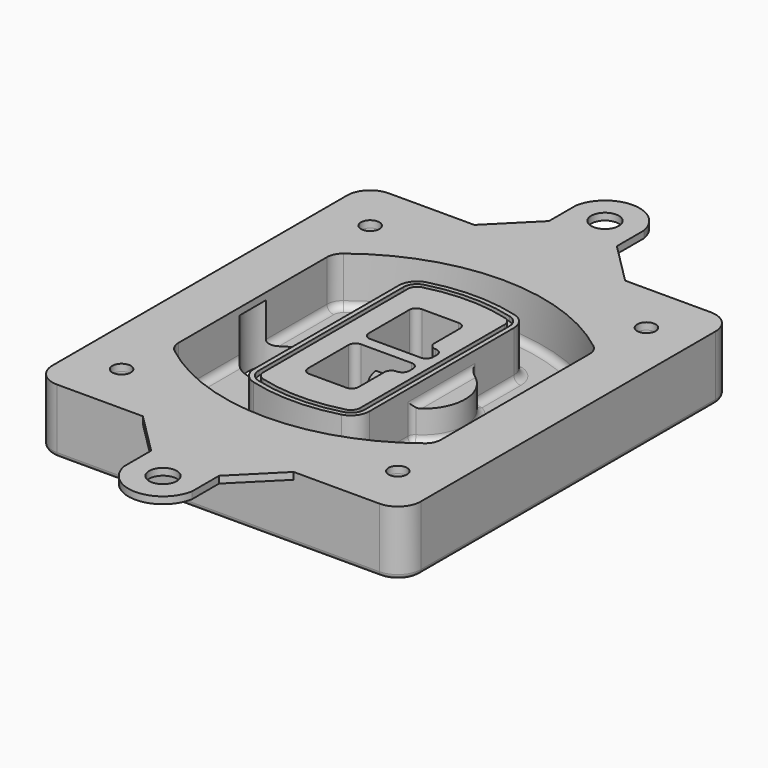
from build123d import *

# Parameters (mm, degrees)
F0_R      = 4
F1_DEPTH  = 25
F2_DEPTH  = 3
F3_DEPTH  = 18
F5_DEPTH  = 21
F6_DEPTH  = 2
F8_DEPTH  = 20
F9_DEPTH  = 16
F10_DEPTH = 25
F7_R      = 6
F7_R_2    = 4
F11_DEPTH = 6
F13_DEPTH = 9
F14_R     = 3
F15_R     = 2
F16_R     = 4
F16_R_2   = 6
F17_DEPTH = 3


# Not quite as in the source:
# - a feature names something its author has since deleted; it is built from what else it names


with BuildPart() as f1:
    # F0 (on Top) → F1 (new body)
    with BuildSketch(Plane.XY):
        with BuildLine():
            ThreePointArc((-80, -80), (-77.0710678119, -87.0710678119), (-70, -90))
            Line((-70, -90), (70, -90))
            ThreePointArc((70, -90), (77.0710678119, -87.0710678119), (80, -80))
            Line((80, -80), (80, 80))
            ThreePointArc((80, 80), (77.0710678119, 87.0710678119), (70, 90))
            Line((70, 90), (-70, 90))
            ThreePointArc((-70, 90), (-77.0710678119, 87.0710678119), (-80, 80))
            Line((-80, 80), (-80, -80))
        make_face()
        with Locations((-60, -67.5)):
            Circle(F0_R, mode=Mode.SUBTRACT)
        with Locations((60, -67.5)):
            Circle(F0_R, mode=Mode.SUBTRACT)
        with Locations((-60, 67.5)):
            Circle(F0_R, mode=Mode.SUBTRACT)
        with BuildLine():
            ThreePointArc((-64, 40.2934422872), (-62.5820384798, 46.4328484224), (-58.6153846154, 51.3286200352))
            ThreePointArc((-58.6153846154, 51.3286200352), (0, 71.5), (58.6153846154, 51.3286200352))
            ThreePointArc((58.6153846154, 51.3286200352), (62.5820384798, 46.4328484224), (64, 40.2934422872))
            Line((64, 40.2934422872), (64, -40.2934422872))
            ThreePointArc((64, -40.2934422872), (62.5820384798, -46.4328484224), (58.6153846154, -51.3286200352))
            ThreePointArc((58.6153846154, -51.3286200352), (0, -71.5), (-58.6153846154, -51.3286200352))
            ThreePointArc((-58.6153846154, -51.3286200352), (-62.5820384798, -46.4328484224), (-64, -40.2934422872))
            Line((-64, -40.2934422872), (-64, 40.2934422872))
        make_face(mode=Mode.SUBTRACT)
        with Locations((60, 67.5)):
            Circle(F0_R, mode=Mode.SUBTRACT)
        with BuildLine():
            ThreePointArc((58.6153846154, 51.3286200352), (0, 71.5), (-58.6153846154, 51.3286200352))
            ThreePointArc((-58.6153846154, 51.3286200352), (-62.5820384798, 46.4328484224), (-64, 40.2934422872))
            Line((-64, 40.2934422872), (-64, -40.2934422872))
            ThreePointArc((-64, -40.2934422872), (-62.5820384798, -46.4328484224), (-58.6153846154, -51.3286200352))
            ThreePointArc((-58.6153846154, -51.3286200352), (0, -71.5), (58.6153846154, -51.3286200352))
            ThreePointArc((58.6153846154, -51.3286200352), (62.5820384798, -46.4328484224), (64, -40.2934422872))
            Line((64, -40.2934422872), (64, 40.2934422872))
            ThreePointArc((64, 40.2934422872), (62.5820384798, 46.4328484224), (58.6153846154, 51.3286200352))
        make_face()
        with BuildLine():
            Line((-60, -40.2934422872), (-60, 40.2934422872))
            ThreePointArc((-60, 40.2934422872), (-58.9871703427, 44.6787323838), (-56.1538461538, 48.1757121072))
            ThreePointArc((-56.1538461538, 48.1757121072), (0, 67.5), (56.1538461538, 48.1757121072))
            ThreePointArc((56.1538461538, 48.1757121072), (58.9871703427, 44.6787323838), (60, 40.2934422872))
            Line((60, 40.2934422872), (60, -40.2934422872))
            ThreePointArc((60, -40.2934422872), (58.9871703427, -44.6787323838), (56.1538461538, -48.1757121072))
            ThreePointArc((56.1538461538, -48.1757121072), (0, -67.5), (-56.1538461538, -48.1757121072))
            ThreePointArc((-56.1538461538, -48.1757121072), (-58.9871703427, -44.6787323838), (-60, -40.2934422872))
        make_face(mode=Mode.SUBTRACT)
        with BuildLine():
            ThreePointArc((-56.1538461538, 48.1757121072), (-58.9871703427, 44.6787323838), (-60, 40.2934422872))
            Line((-60, 40.2934422872), (-60, -40.2934422872))
            ThreePointArc((-60, -40.2934422872), (-58.9871703427, -44.6787323838), (-56.1538461538, -48.1757121072))
            ThreePointArc((-56.1538461538, -48.1757121072), (0, -67.5), (56.1538461538, -48.1757121072))
            ThreePointArc((56.1538461538, -48.1757121072), (58.9871703427, -44.6787323838), (60, -40.2934422872))
            Line((60, -40.2934422872), (60, 40.2934422872))
            ThreePointArc((60, 40.2934422872), (58.9871703427, 44.6787323838), (56.1538461538, 48.1757121072))
            ThreePointArc((56.1538461538, 48.1757121072), (0, 67.5), (-56.1538461538, 48.1757121072))
        make_face()
        with BuildLine():
            ThreePointArc((54.3076923077, 45.8110311612), (56.2910192399, 43.3631453548), (57, 40.2934422872))
            Line((57, 40.2934422872), (57, -40.2934422872))
            ThreePointArc((57, -40.2934422872), (56.2910192399, -43.3631453548), (54.3076923077, -45.8110311612))
            ThreePointArc((54.3076923077, -45.8110311612), (0, -64.5), (-54.3076923077, -45.8110311612))
            ThreePointArc((-54.3076923077, -45.8110311612), (-56.2910192399, -43.3631453548), (-57, -40.2934422872))
            Line((-57, -40.2934422872), (-57, 40.2934422872))
            ThreePointArc((-57, 40.2934422872), (-56.2910192399, 43.3631453548), (-54.3076923077, 45.8110311612))
            ThreePointArc((-54.3076923077, 45.8110311612), (0, 64.5), (54.3076923077, 45.8110311612))
        make_face(mode=Mode.SUBTRACT)
        with BuildLine():
            Line((57, -40.2934422872), (57, 40.2934422872))
            ThreePointArc((57, 40.2934422872), (56.2910192399, 43.3631453548), (54.3076923077, 45.8110311612))
            ThreePointArc((54.3076923077, 45.8110311612), (0, 64.5), (-54.3076923077, 45.8110311612))
            ThreePointArc((-54.3076923077, 45.8110311612), (-56.2910192399, 43.3631453548), (-57, 40.2934422872))
            Line((-57, 40.2934422872), (-57, -40.2934422872))
            ThreePointArc((-57, -40.2934422872), (-56.2910192399, -43.3631453548), (-54.3076923077, -45.8110311612))
            ThreePointArc((-54.3076923077, -45.8110311612), (0, -64.5), (54.3076923077, -45.8110311612))
            ThreePointArc((54.3076923077, -45.8110311612), (56.2910192399, -43.3631453548), (57, -40.2934422872))
        make_face()
    extrude(amount=-F1_DEPTH)

    # F0 (on Top) → F2 (join)
    with BuildSketch(Plane.XY):
        with BuildLine():
            ThreePointArc((-56.1538461538, 48.1757121072), (-58.9871703427, 44.6787323838), (-60, 40.2934422872))
            Line((-60, 40.2934422872), (-60, -40.2934422872))
            ThreePointArc((-60, -40.2934422872), (-58.9871703427, -44.6787323838), (-56.1538461538, -48.1757121072))
            ThreePointArc((-56.1538461538, -48.1757121072), (0, -67.5), (56.1538461538, -48.1757121072))
            ThreePointArc((56.1538461538, -48.1757121072), (58.9871703427, -44.6787323838), (60, -40.2934422872))
            Line((60, -40.2934422872), (60, 40.2934422872))
            ThreePointArc((60, 40.2934422872), (58.9871703427, 44.6787323838), (56.1538461538, 48.1757121072))
            ThreePointArc((56.1538461538, 48.1757121072), (0, 67.5), (-56.1538461538, 48.1757121072))
        make_face()
        with BuildLine():
            ThreePointArc((54.3076923077, 45.8110311612), (56.2910192399, 43.3631453548), (57, 40.2934422872))
            Line((57, 40.2934422872), (57, -40.2934422872))
            ThreePointArc((57, -40.2934422872), (56.2910192399, -43.3631453548), (54.3076923077, -45.8110311612))
            ThreePointArc((54.3076923077, -45.8110311612), (0, -64.5), (-54.3076923077, -45.8110311612))
            ThreePointArc((-54.3076923077, -45.8110311612), (-56.2910192399, -43.3631453548), (-57, -40.2934422872))
            Line((-57, -40.2934422872), (-57, 40.2934422872))
            ThreePointArc((-57, 40.2934422872), (-56.2910192399, 43.3631453548), (-54.3076923077, 45.8110311612))
            ThreePointArc((-54.3076923077, 45.8110311612), (0, 64.5), (54.3076923077, 45.8110311612))
        make_face(mode=Mode.SUBTRACT)
    extrude(amount=F2_DEPTH)

    # F0 (on Top) → F3 (cut)
    with BuildSketch(Plane.XY):
        with BuildLine():
            Line((57, -40.2934422872), (57, 40.2934422872))
            ThreePointArc((57, 40.2934422872), (56.2910192399, 43.3631453548), (54.3076923077, 45.8110311612))
            ThreePointArc((54.3076923077, 45.8110311612), (0, 64.5), (-54.3076923077, 45.8110311612))
            ThreePointArc((-54.3076923077, 45.8110311612), (-56.2910192399, 43.3631453548), (-57, 40.2934422872))
            Line((-57, 40.2934422872), (-57, -40.2934422872))
            ThreePointArc((-57, -40.2934422872), (-56.2910192399, -43.3631453548), (-54.3076923077, -45.8110311612))
            ThreePointArc((-54.3076923077, -45.8110311612), (0, -64.5), (54.3076923077, -45.8110311612))
            ThreePointArc((54.3076923077, -45.8110311612), (56.2910192399, -43.3631453548), (57, -40.2934422872))
        make_face()
    extrude(amount=-F3_DEPTH, mode=Mode.SUBTRACT)

    # F4 (on face) → F5 (join, through all)
    with BuildSketch(Plane.XY.offset(3)):
        with BuildLine():
            ThreePointArc((-25, -39.2465276821), (-23.3511545998, -44.1109737193), (-19.0842911877, -46.9702398883))
            ThreePointArc((-19.0842911877, -46.9702398883), (0, -49.5), (19.0842911877, -46.9702398883))
            ThreePointArc((19.0842911877, -46.9702398883), (23.3511545998, -44.1109737193), (25, -39.2465276821))
            Line((25, -39.2465276821), (25, 39.2465276821))
            ThreePointArc((25, 39.2465276821), (23.3511545998, 44.1109737193), (19.0842911877, 46.9702398883))
            ThreePointArc((19.0842911877, 46.9702398883), (0, 49.5), (-19.0842911877, 46.9702398883))
            ThreePointArc((-19.0842911877, 46.9702398883), (-23.3511545998, 44.1109737193), (-25, 39.2465276821))
            Line((-25, 39.2465276821), (-25, -39.2465276821))
        make_face()
        with BuildLine():
            ThreePointArc((18.5632183908, 45.0393118368), (21.7633659499, 42.89486221), (23, 39.2465276821))
            Line((23, 39.2465276821), (23, -39.2465276821))
            ThreePointArc((23, -39.2465276821), (21.7633659499, -42.89486221), (18.5632183908, -45.0393118368))
            ThreePointArc((18.5632183908, -45.0393118368), (0, -47.5), (-18.5632183908, -45.0393118368))
            ThreePointArc((-18.5632183908, -45.0393118368), (-21.7633659499, -42.89486221), (-23, -39.2465276821))
            Line((-23, -39.2465276821), (-23, 39.2465276821))
            ThreePointArc((-23, 39.2465276821), (-21.7633659499, 42.89486221), (-18.5632183908, 45.0393118368))
            ThreePointArc((-18.5632183908, 45.0393118368), (0, 47.5), (18.5632183908, 45.0393118368))
        make_face(mode=Mode.SUBTRACT)
        with BuildLine():
            Line((23, -39.2465276821), (23, 39.2465276821))
            ThreePointArc((23, 39.2465276821), (21.7633659499, 42.89486221), (18.5632183908, 45.0393118368))
            ThreePointArc((18.5632183908, 45.0393118368), (0, 47.5), (-18.5632183908, 45.0393118368))
            ThreePointArc((-18.5632183908, 45.0393118368), (-21.7633659499, 42.89486221), (-23, 39.2465276821))
            Line((-23, 39.2465276821), (-23, -39.2465276821))
            ThreePointArc((-23, -39.2465276821), (-21.7633659499, -42.89486221), (-18.5632183908, -45.0393118368))
            ThreePointArc((-18.5632183908, -45.0393118368), (0, -47.5), (18.5632183908, -45.0393118368))
            ThreePointArc((18.5632183908, -45.0393118368), (21.7633659499, -42.89486221), (23, -39.2465276821))
        make_face()
        with BuildLine():
            ThreePointArc((18.0421455939, 43.1083837852), (20.1755772999, 41.6787507007), (21, 39.2465276821))
            Line((21, 39.2465276821), (21, -39.2465276821))
            ThreePointArc((21, -39.2465276821), (20.1755772999, -41.6787507007), (18.0421455939, -43.1083837852))
            ThreePointArc((18.0421455939, -43.1083837852), (0, -45.5), (-18.0421455939, -43.1083837852))
            ThreePointArc((-18.0421455939, -43.1083837852), (-20.1755772999, -41.6787507007), (-21, -39.2465276821))
            Line((-21, -39.2465276821), (-21, 39.2465276821))
            ThreePointArc((-21, 39.2465276821), (-20.1755772999, 41.6787507007), (-18.0421455939, 43.1083837852))
            ThreePointArc((-18.0421455939, 43.1083837852), (0, 45.5), (18.0421455939, 43.1083837852))
        make_face(mode=Mode.SUBTRACT)
        with BuildLine():
            Line((21, -39.2465276821), (21, 39.2465276821))
            ThreePointArc((21, 39.2465276821), (20.1755772999, 41.6787507007), (18.0421455939, 43.1083837852))
            ThreePointArc((18.0421455939, 43.1083837852), (0, 45.5), (-18.0421455939, 43.1083837852))
            ThreePointArc((-18.0421455939, 43.1083837852), (-20.1755772999, 41.6787507007), (-21, 39.2465276821))
            Line((-21, 39.2465276821), (-21, -39.2465276821))
            ThreePointArc((-21, -39.2465276821), (-20.1755772999, -41.6787507007), (-18.0421455939, -43.1083837852))
            ThreePointArc((-18.0421455939, -43.1083837852), (0, -45.5), (18.0421455939, -43.1083837852))
            ThreePointArc((18.0421455939, -43.1083837852), (20.1755772999, -41.6787507007), (21, -39.2465276821))
        make_face()
        with BuildLine():
            Line((-8, -2.5), (14, -2.5))
            ThreePointArc((14, -2.5), (16.1213203436, -3.3786796564), (17, -5.5))
            Line((17, -5.5), (17, -7.5))
            ThreePointArc((17, -7.5), (16.1213203436, -9.6213203436), (14, -10.5))
            ThreePointArc((14, -10.5), (11.8786796564, -11.3786796564), (11, -13.5))
            Line((11, -13.5), (11, -27.5))
            ThreePointArc((11, -27.5), (10.1213203436, -29.6213203436), (8, -30.5))
            Line((8, -30.5), (-8, -30.5))
            ThreePointArc((-8, -30.5), (-10.1213203436, -29.6213203436), (-11, -27.5))
            Line((-11, -27.5), (-11, -5.5))
            ThreePointArc((-11, -5.5), (-10.1213203436, -3.3786796564), (-8, -2.5))
        make_face(mode=Mode.SUBTRACT)
        with BuildLine():
            ThreePointArc((-8, 2.5), (-10.1213203436, 3.3786796564), (-11, 5.5))
            Line((-11, 5.5), (-11, 27.5))
            ThreePointArc((-11, 27.5), (-10.1213203436, 29.6213203436), (-8, 30.5))
            Line((-8, 30.5), (8, 30.5))
            ThreePointArc((8, 30.5), (10.1213203436, 29.6213203436), (11, 27.5))
            Line((11, 27.5), (11, 13.5))
            ThreePointArc((11, 13.5), (11.8786796564, 11.3786796564), (14, 10.5))
            ThreePointArc((14, 10.5), (16.1213203436, 9.6213203436), (17, 7.5))
            Line((17, 7.5), (17, 5.5))
            ThreePointArc((17, 5.5), (16.1213203436, 3.3786796564), (14, 2.5))
            Line((14, 2.5), (-8, 2.5))
        make_face(mode=Mode.SUBTRACT)
    extrude(amount=-F5_DEPTH)

    # F4 (on face) → F6 (cut)
    with BuildSketch(Plane.XY.offset(3)):
        with BuildLine():
            Line((23, -39.2465276821), (23, 39.2465276821))
            ThreePointArc((23, 39.2465276821), (21.7633659499, 42.89486221), (18.5632183908, 45.0393118368))
            ThreePointArc((18.5632183908, 45.0393118368), (0, 47.5), (-18.5632183908, 45.0393118368))
            ThreePointArc((-18.5632183908, 45.0393118368), (-21.7633659499, 42.89486221), (-23, 39.2465276821))
            Line((-23, 39.2465276821), (-23, -39.2465276821))
            ThreePointArc((-23, -39.2465276821), (-21.7633659499, -42.89486221), (-18.5632183908, -45.0393118368))
            ThreePointArc((-18.5632183908, -45.0393118368), (0, -47.5), (18.5632183908, -45.0393118368))
            ThreePointArc((18.5632183908, -45.0393118368), (21.7633659499, -42.89486221), (23, -39.2465276821))
        make_face()
        with BuildLine():
            ThreePointArc((18.0421455939, 43.1083837852), (20.1755772999, 41.6787507007), (21, 39.2465276821))
            Line((21, 39.2465276821), (21, -39.2465276821))
            ThreePointArc((21, -39.2465276821), (20.1755772999, -41.6787507007), (18.0421455939, -43.1083837852))
            ThreePointArc((18.0421455939, -43.1083837852), (0, -45.5), (-18.0421455939, -43.1083837852))
            ThreePointArc((-18.0421455939, -43.1083837852), (-20.1755772999, -41.6787507007), (-21, -39.2465276821))
            Line((-21, -39.2465276821), (-21, 39.2465276821))
            ThreePointArc((-21, 39.2465276821), (-20.1755772999, 41.6787507007), (-18.0421455939, 43.1083837852))
            ThreePointArc((-18.0421455939, 43.1083837852), (0, 45.5), (18.0421455939, 43.1083837852))
        make_face(mode=Mode.SUBTRACT)
    extrude(amount=-F6_DEPTH, mode=Mode.SUBTRACT)

    # F7 (on face) → F8 (join)
    with BuildSketch(Plane(origin=(0, 0, -25), x_dir=(1, 0, 0), z_dir=(0, 0, -1))):
        with BuildLine():
            ThreePointArc((3.28842436, 0), (16.7567035675, 13.4682792075), (30.224982775, 0))
            Line((30.224982775, 0), (35.224982775, 0))
            ThreePointArc((35.224982775, 0), (16.7567035675, 18.4682792075), (-1.71157564, 0))
            Line((-1.71157564, 0), (3.28842436, 0))
        make_face()
        with BuildLine():
            Line((3.28842436, 0), (30.224982775, 0))
            ThreePointArc((30.224982775, 0), (16.7567035675, 13.4682792075), (3.28842436, 0))
        make_face()
        with BuildLine():
            ThreePointArc((3.28842436, 0), (16.7567035675, -13.4682792075), (30.224982775, 0))
            Line((30.224982775, 0), (3.28842436, 0))
        make_face()
        with BuildLine():
            Line((35.224982775, 0), (30.224982775, 0))
            ThreePointArc((30.224982775, 0), (16.7567035675, -13.4682792075), (3.28842436, 0))
            Line((3.28842436, 0), (-1.71157564, 0))
            ThreePointArc((-1.71157564, 0), (16.7567035675, -18.4682792075), (35.224982775, 0))
        make_face()
    extrude(amount=-F8_DEPTH)

    # F7 (on face) → F9 (cut)
    with BuildSketch(Plane(origin=(0, 0, -25), x_dir=(1, 0, 0), z_dir=(0, 0, -1))):
        with BuildLine():
            Line((3.28842436, 0), (30.224982775, 0))
            ThreePointArc((30.224982775, 0), (16.7567035675, 13.4682792075), (3.28842436, 0))
        make_face()
        with BuildLine():
            ThreePointArc((3.28842436, 0), (16.7567035675, -13.4682792075), (30.224982775, 0))
            Line((30.224982775, 0), (3.28842436, 0))
        make_face()
    extrude(amount=-F9_DEPTH, mode=Mode.SUBTRACT)

    # F7 (on face) → F10 (cut)
    with BuildSketch(Plane(origin=(0, 0, -25), x_dir=(1, 0, 0), z_dir=(0, 0, -1))):
        with BuildLine():
            Line((-59.0318229325, 0), (-32.0952645175, 0))
            ThreePointArc((-32.0952645175, 0), (-45.563543725, 13.4682792075), (-59.0318229325, 0))
        make_face()
        with BuildLine():
            ThreePointArc((-59.0318229325, 0), (-45.563543725, -13.4682792075), (-32.0952645175, 0))
            Line((-32.0952645175, 0), (-59.0318229325, 0))
        make_face()
    extrude(amount=-F10_DEPTH, mode=Mode.SUBTRACT)

    # F7 (on face) → F11 (cut)
    with BuildSketch(Plane(origin=(0, 0, -25), x_dir=(1, 0, 0), z_dir=(0, 0, -1))):
        with Locations((60, -67.5)):
            Circle(F7_R)
        with Locations((60, -67.5)):
            Circle(F7_R_2, mode=Mode.SUBTRACT)
        with Locations((-60, -67.5)):
            Circle(F7_R)
        with Locations((-60, -67.5)):
            Circle(F7_R_2, mode=Mode.SUBTRACT)
        with Locations((-60, 67.5)):
            Circle(F7_R)
        with Locations((-60, 67.5)):
            Circle(F7_R_2, mode=Mode.SUBTRACT)
        with Locations((60, 67.5)):
            Circle(F7_R)
        with Locations((60, 67.5)):
            Circle(F7_R_2, mode=Mode.SUBTRACT)
    extrude(amount=-F11_DEPTH, mode=Mode.SUBTRACT)

    # F12 (on face) → F13 (cut, through all)
    with BuildSketch(Plane(origin=(0, 0, -9), x_dir=(1, 0, 0), z_dir=(0, 0, -1))):
        with BuildLine():
            Line((11, 13.5), (11, 17.5481537753))
            ThreePointArc((11, 17.5481537753), (2.5696536419, 11.8239143813), (-1.5415842455, 2.5))
            Line((-1.5415842455, 2.5), (3.5224848595, 2.5))
            ThreePointArc((3.5224848595, 2.5), (6.1857188154, 8.3455872281), (11.2536447004, 12.2927168648))
            ThreePointArc((11.2536447004, 12.2927168648), (11.0640958889, 12.8831798879), (11, 13.5))
        make_face()
        with BuildLine():
            ThreePointArc((11.2536447004, -12.2927168648), (6.1857188154, -8.3455872281), (3.5224848595, -2.5))
            Line((3.5224848595, -2.5), (-1.5415842455, -2.5))
            ThreePointArc((-1.5415842455, -2.5), (2.5696536419, -11.8239143813), (11, -17.5481537753))
            Line((11, -17.5481537753), (11, -13.5))
            ThreePointArc((11, -13.5), (11.0640958889, -12.8831798879), (11.2536447004, -12.2927168648))
        make_face()
        with BuildLine():
            ThreePointArc((11.2536447004, 12.2927168648), (6.1857188154, 8.3455872281), (3.5224848595, 2.5))
            Line((3.5224848595, 2.5), (14, 2.5))
            ThreePointArc((14, 2.5), (16.1213203436, 3.3786796564), (17, 5.5))
            Line((17, 5.5), (17, 7.5))
            ThreePointArc((17, 7.5), (16.1213203436, 9.6213203436), (14, 10.5))
            ThreePointArc((14, 10.5), (12.3601599782, 10.9878446101), (11.2536447004, 12.2927168648))
        make_face()
        with BuildLine():
            Line((14, -2.5), (3.5224848595, -2.5))
            ThreePointArc((3.5224848595, -2.5), (6.1857188154, -8.3455872281), (11.2536447004, -12.2927168648))
            ThreePointArc((11.2536447004, -12.2927168648), (12.3601599782, -10.9878446101), (14, -10.5))
            ThreePointArc((14, -10.5), (16.1213203436, -9.6213203436), (17, -7.5))
            Line((17, -7.5), (17, -5.5))
            ThreePointArc((17, -5.5), (16.1213203436, -3.3786796564), (14, -2.5))
        make_face()
    extrude(amount=F13_DEPTH, mode=Mode.SUBTRACT)

    # F14
    f14_edges = [f1.edges().sort_by_distance(p)[0] for p in [
        (-57, -23.703476, -18),
        (-57, 23.703476, -18),
        (25, 0, -5),
        (25, 16.526506, -11.5),
        (25, -16.526506, -11.5),
        (25, -27.886517, -18),
        (35.224983, 0, -18),
    ]]
    fillet(f14_edges, radius=F14_R)

    # F15
    f15_edges = [f1.edges().sort_by_distance(p)[0] for p in [
        (0, -90, -25),
    ]]
    fillet(f15_edges, radius=F15_R)

    # F16 (on face) → F17 (join, through all)
    with BuildSketch(Plane.XY):
        with BuildLine():
            Line((-32.7464278423, 90), (-70, 90))
            ThreePointArc((-70, 90), (-77.0710678119, 87.0710678119), (-80, 80))
            Line((-80, 80), (-80, -80))
            ThreePointArc((-80, -80), (-77.0710678119, -87.0710678119), (-70, -90))
            Line((-70, -90), (-32.7464278423, -90))
            Line((-32.7464278423, -90), (32.7464278423, -90))
            Line((32.7464278423, -90), (70, -90))
            ThreePointArc((70, -90), (77.0710678119, -87.0710678119), (80, -80))
            Line((80, -80), (80, 80))
            ThreePointArc((80, 80), (77.0710678119, 87.0710678119), (70, 90))
            Line((70, 90), (32.7464278423, 90))
            Line((32.7464278423, 90), (-32.7464278423, 90))
        make_face()
        with Locations((-60, -67.5)):
            Circle(F16_R, mode=Mode.SUBTRACT)
        with Locations((60, -67.5)):
            Circle(F16_R, mode=Mode.SUBTRACT)
        with Locations((-60, 67.5)):
            Circle(F16_R, mode=Mode.SUBTRACT)
        with BuildLine():
            ThreePointArc((56.1538461538, 48.1757121072), (58.9871703427, 44.6787323838), (60, 40.2934422872))
            Line((60, 40.2934422872), (60, -40.2934422872))
            ThreePointArc((60, -40.2934422872), (58.9871703427, -44.6787323838), (56.1538461538, -48.1757121072))
            ThreePointArc((56.1538461538, -48.1757121072), (0, -67.5), (-56.1538461538, -48.1757121072))
            ThreePointArc((-56.1538461538, -48.1757121072), (-58.9871703427, -44.6787323838), (-60, -40.2934422872))
            Line((-60, -40.2934422872), (-60, 40.2934422872))
            ThreePointArc((-60, 40.2934422872), (-58.9871703427, 44.6787323838), (-56.1538461538, 48.1757121072))
            ThreePointArc((-56.1538461538, 48.1757121072), (0, 67.5), (56.1538461538, 48.1757121072))
        make_face(mode=Mode.SUBTRACT)
        with Locations((60, 67.5)):
            Circle(F16_R, mode=Mode.SUBTRACT)
        with BuildLine():
            Line((-14.7464278423, 108), (-32.7464278423, 90))
            Line((-32.7464278423, 90), (32.7464278423, 90))
            Line((32.7464278423, 90), (14.7464278423, 108))
            Line((14.7464278423, 108), (14.7464278423, 122.7464278423))
            ThreePointArc((14.7464278423, 122.7464278423), (0, 135), (-14.7464278423, 122.7464278423))
            Line((-14.7464278423, 122.7464278423), (-14.7464278423, 108))
        make_face()
        with Locations((0, 120)):
            Circle(F16_R_2, mode=Mode.SUBTRACT)
        with BuildLine():
            Line((32.7464278423, -90), (-32.7464278423, -90))
            Line((-32.7464278423, -90), (-14.7464278423, -108))
            Line((-14.7464278423, -108), (-14.7464278423, -122.7464278423))
            ThreePointArc((-14.7464278423, -122.7464278423), (0, -135), (14.7464278423, -122.7464278423))
            Line((14.7464278423, -122.7464278423), (14.7464278423, -108))
            Line((14.7464278423, -108), (32.7464278423, -90))
        make_face()
        with Locations((0, -120)):
            Circle(F16_R_2, mode=Mode.SUBTRACT)
    extrude(amount=F17_DEPTH)


solid = f1.part
